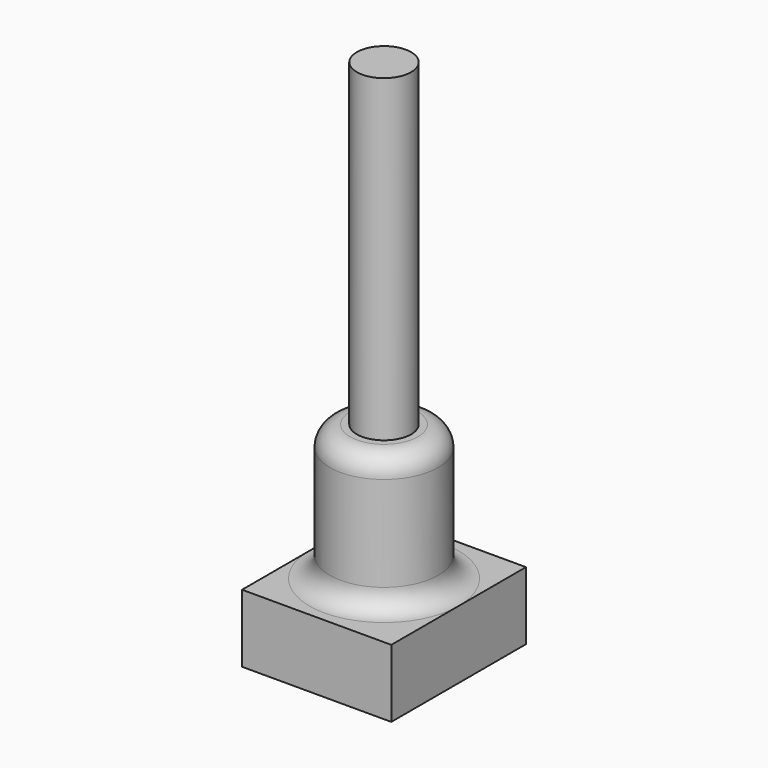
from build123d import *

# Parameters (mm, degrees)
F0_W     = 22
F0_H     = 24.8139590786
F1_DEPTH = 10
F2_R     = 8
F3_DEPTH = 20
F4_R     = 4
F5_DEPTH = 47
F6_R     = 2.99999


# Not quite as in the source:
# - a fillet or chamfer is up to 0.001 mm smaller than in the source, because OpenCascade refuses the exact size


with BuildPart() as f1:
    # F0 (on Top) → F1 (new body)
    with BuildSketch(Plane.XY):
        Rectangle(F0_W, F0_H)
    extrude(amount=F1_DEPTH)

    # F2 (on face) → F3 (join)
    with BuildSketch(Plane.XY.offset(10)):
        Circle(F2_R)
    extrude(amount=F3_DEPTH)

    # F4 (on face) → F5 (join)
    with BuildSketch(Plane.XY.offset(30)):
        Circle(F4_R)
    extrude(amount=F5_DEPTH)

    # F6 (radius 3 in the source; OpenCascade refuses exactly that, so slightly less here)
    f6_edges = [f1.edges().sort_by_distance(p)[0] for p in [
        (8, 0, 20),
        (-8, 0, 10),
        (-8, 0, 30),
    ]]
    fillet(f6_edges, radius=F6_R)


solid = f1.part
